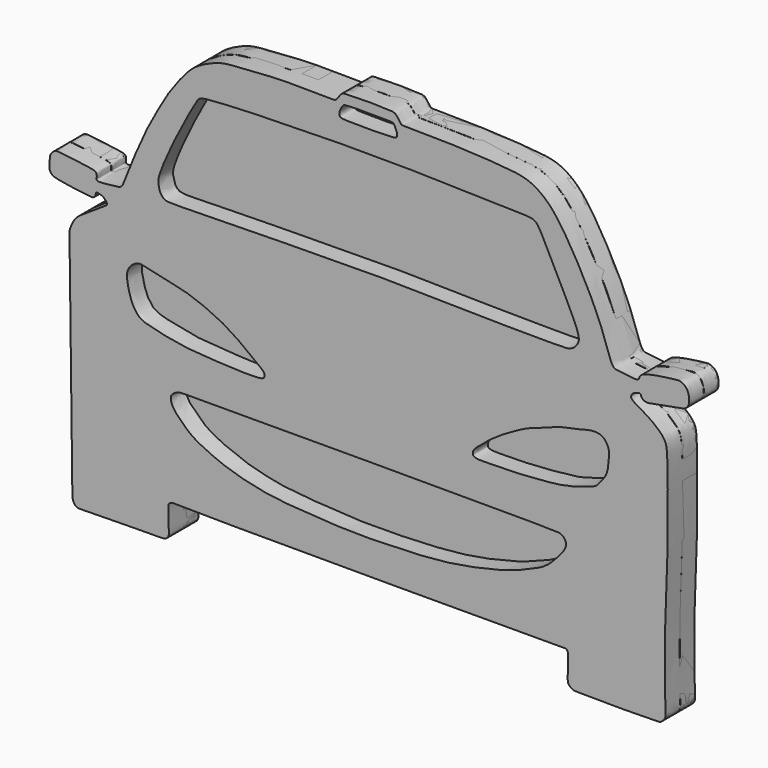
from build123d import *

# Parameters (mm, degrees)
F1_DEPTH = 10
F3_DEPTH = 5


# Not quite as in the source:
# - the dataset's text gives a spline's control points without its knots; the knots are read off the source's solid


with BuildPart() as f1:
    # F0 (on Front) → F1 (new body)
    with BuildSketch(Plane.XZ):
        with BuildLine():
            add(Edge.make_bspline(
                [(-21.2726220489, 56.9635778666), (-18.9281210434, 56.9386434726), (-13.6200187911, 56.9350553762), (-12.4767039382, 56.8796603206), (-11.0844689446, 59.0635225696), (-10.0407495433, 59.5178063954), (2.4345859918, 59.518579453), (3.2763047499, 59.1466182179), (3.9763116908, 58.8890525048), (5.0929181479, 56.9335783544), (5.904101681, 56.724426004), (15.4186256689, 56.7606694424), (22.415242163, 56.5636878104), (29.6627233817, 56.1516039707), (36.4134224992, 55.6653181625), (40.7970991211, 54.6157339048), (45.7371435577, 51.1119020349), (50.2355062798, 44.586092306), (55.3245831337, 35.7107979243), (59.9788649432, 25.7843744812), (62.2274911548, 17.8785094194), (63.6873972743, 17.2156075688), (66.8512747735, 16.9837572481), (69.6520031247, 16.5690870165), (69.8806873946, 17.6725077821), (70.4097864802, 18.6062553039), (74.7105095588, 19.635285385), (79.2407912013, 20.1558018394), (81.1270530867, 20.4040771455), (82.9879359908, 19.1249872852), (83.5930078541, 16.4735751448), (82.9736764331, 13.9928114241), (79.4258491754, 13.6783873856), (73.7801155733, 12.3750310277), (71.463650212, 12.0317762657), (70.2694302292, 12.9854799945), (70.3246556827, 14.0053639175), (68.0167941293, 13.3915679245), (67.2779003031, 11.8146832667), (69.6477321499, 10.3935148412), (73.5277584139, 8.2297653036), (76.3688101278, 5.512225397), (77.553760652, 3.3461910931), (77.5530453586, -6.9270704509), (77.6729301989, -20.5721617917), (76.8765812567, -35.8181398753), (76.7627137917, -48.5519759849), (76.7695297304, -57.1100262171), (77.1198420733, -60.9187955099), (76.7184740375, -61.9661008778), (75.7188165531, -62.9575649684), (74.57226928, -63.2191940943), (52.313578017, -63.2602932478), (51.7170076075, -62.9598727868), (50.8037103143, -62.3515989217), (50.4461995219, -61.6734356735), (50.3566400858, -60.312061393), (50.496949856, -55.8709343448), (50.5163145323, -54.6497774244), (50.2924540607, -53.7307567814), (48.869529547, -53.7163267319), (48.4763551332, -53.8276018998), (-54.7929577116, -54.0161919263), (-56.6230034085, -53.5809102698), (-57.8696673343, -53.9463225485), (-57.9690717545, -54.8661327531), (-57.9613761424, -55.8743450215), (-57.78340253, -61.3734469783), (-57.906912999, -61.8656330337), (-58.3760760652, -62.8292128086), (-59.8541306513, -63.0064316834), (-61.119934638, -62.9784770213), (-81.3057995002, -63.1510879072), (-81.9270637775, -63.3194642105), (-83.0199574255, -63.1533789577), (-83.5677741934, -62.4923589555), (-84.0399677683, -61.4612616226), (-84.1109783652, -59.7084531519), (-84.0532967239, -54.3188819205), (-84.2059386301, -39.499846326), (-84.5404697297, -24.4846736289), (-84.6842054736, -4.2904268447), (-84.9727713877, 1.6036548675), (-84.6122092098, 3.1704690828), (-83.4970696269, 5.5484038074), (-81.9083921978, 6.9864352173), (-78.9297296369, 8.7724944135), (-76.6131468274, 10.515826782), (-74.6581214491, 11.5553240796), (-74.6426954546, 12.1225788132), (-75.0666632198, 12.9146555158), (-76.0348664394, 13.591346412), (-77.0102810448, 13.8064368612), (-77.5889687922, 13.8905870458), (-77.7555570585, 13.1194908993), (-77.8783275013, 12.5728149948), (-78.6488107317, 12.2151925415), (-79.8144730652, 12.3421801098), (-87.754645938, 13.3273577072), (-89.7442692365, 14.0688538765), (-90.3708386486, 15.3126490716), (-90.2186233578, 16.685187407), (-90.2011514391, 18.346575344), (-89.7260237086, 19.3326468169), (-88.6939660926, 20.2602979581), (-87.0893708951, 20.1537941529), (-84.2859429545, 19.7755893206), (-80.7326560197, 19.3338400413), (-78.0451968926, 18.9618621225), (-77.4081568708, 18.4038525579), (-77.3850675835, 17.3042629393), (-77.6174256376, 16.6571560893), (-76.0385293662, 16.5012085027), (-73.6413404779, 16.9400882023), (-70.68829264, 16.9931303492), (-70.0675967459, 18.6874870731), (-68.5910153059, 22.5032449084), (-64.2564188952, 32.8703041995), (-60.8249096081, 38.9385754701), (-57.8737837643, 44.1866083784), (-54.2854935401, 48.980022304), (-51.057079458, 52.4849366267), (-47.5395759836, 54.3378193748), (-43.7334971009, 55.8696843536), (-39.8300474742, 56.2378976637), (-32.3869709385, 56.8090194268), (-25.0928653652, 57.0502633666), (-22.9556034711, 56.9814768232), (-21.2726220489, 56.9635778666)],
                knots=[0, 0, 0, 0, 0.012004279, 0.0166060931, 0.0229256448, 0.0281319073, 0.0432673507, 0.0475023634, 0.0509727754, 0.0572163817, 0.0610794225, 0.0740101169, 0.0861690954, 0.0977510892, 0.1089672006, 0.1180487717, 0.1284009233, 0.1405580043, 0.1544730395, 0.1693317649, 0.1811779425, 0.1860858482, 0.1939223982, 0.2008529986, 0.2047123352, 0.2088215587, 0.2178047105, 0.2273021586, 0.2330687556, 0.2391473012, 0.2462002175, 0.2524569245, 0.2602934775, 0.2709255551, 0.2774471417, 0.2823111627, 0.2858315267, 0.2918561735, 0.2968070097, 0.3033862826, 0.3128308377, 0.3212326352, 0.3276933936, 0.3410856773, 0.3575651839, 0.3745816846, 0.3901986349, 0.4028768542, 0.4109320455, 0.4153236614, 0.4199204056, 0.4252759381, 0.4455314568, 0.4496448447, 0.4537977426, 0.4574222191, 0.4625115378, 0.4716783043, 0.4766263187, 0.4803465727, 0.4847295197, 0.4896306962, 0.533369126, 0.5407513134, 0.5447167402, 0.5484229444, 0.5531979597, 0.5632282462, 0.5665861336, 0.5706917749, 0.5754184792, 0.5812469368, 0.6004920236, 0.6046145035, 0.6087124203, 0.6126751413, 0.6171358015, 0.6225679613, 0.63233332, 0.648837342, 0.6664896516, 0.6859542941, 0.6959514414, 0.7011876078, 0.7079812388, 0.7143927888, 0.722400922, 0.7300977008, 0.7361918541, 0.7390107332, 0.7429853976, 0.7477261765, 0.7520874229, 0.7550056805, 0.7585574057, 0.7618058195, 0.7653503812, 0.7701326602, 0.7823994269, 0.7887832793, 0.7934012506, 0.7985126711, 0.8040633285, 0.8085537263, 0.8133764402, 0.8186789388, 0.825980184, 0.8344524837, 0.8414202702, 0.845081123, 0.8495126559, 0.8525366189, 0.8572853902, 0.8644418039, 0.8715383863, 0.8766814644, 0.8853463362, 0.8999599019, 0.9116536105, 0.9221471426, 0.9327623493, 0.9421527591, 0.9507359878, 0.9593353611, 0.9678654751, 0.9798461294, 0.9913828237, 1, 1, 1, 1], degree=3))
        make_face()
        with BuildLine():
            add(Edge.make_bspline(
                [(-53.1355589628, -26.5916269273), (-53.6976261616, -26.5964024078), (-54.7832478549, -26.5807781137), (-56.0233124859, -26.9576088353), (-57.4068308066, -28.0020644289), (-57.3223140239, -29.6697594393), (-56.2385573069, -31.6264394585), (-54.574722627, -33.1702280567), (-51.9418061953, -36.0076064052), (-46.3671903717, -38.7239087732), (-40.4685519219, -41.1333015304), (-30.5424899792, -43.4525625201), (-22.3232735976, -43.9772319436), (-9.2867544557, -44.9236923228), (1.1993285628, -44.6889216672), (10.8839715562, -44.3309053124), (18.6551069165, -43.6032529515), (25.152762993, -42.4398108365), (33.9704603673, -40.491225791), (41.4046227696, -37.4482689073), (45.1840875394, -35.5126166261), (48.7429680129, -31.4913886381), (50.0565149772, -29.5272469574), (49.9175813156, -27.8968660654), (48.7318024113, -26.7300201474), (46.5449775529, -26.4557090204), (23.193318347, -26.5842552421), (9.0526969316, -26.3970421968), (-18.087431957, -26.564441631), (-43.2680076928, -26.5233169993), (-50.7705705235, -26.5249350214), (-52.5033477422, -26.5862554834), (-53.1355589628, -26.5916269273)],
                knots=[0, 0, 0, 0, 0.0171126114, 0.0323888607, 0.0490571733, 0.0654263189, 0.0851073726, 0.1051342912, 0.1311088377, 0.1640384324, 0.1984074172, 0.2404194754, 0.2795803906, 0.327564471, 0.3715811823, 0.4130663176, 0.4500873651, 0.4843764852, 0.5249027849, 0.5626102853, 0.5904227705, 0.6209881894, 0.6412442562, 0.6572639193, 0.6729750723, 0.6916365136, 0.754333791, 0.8082138255, 0.8780108631, 0.9459992677, 0.9807517945, 1, 1, 1, 1], degree=3))
        make_face(mode=Mode.SUBTRACT)
        with BuildLine():
            add(Edge.make_bspline(
                [(-69.1952109337, -3.0402038246), (-69.1424189669, -2.4984055481), (-68.8148194617, -1.2736033989), (-67.3949290593, 0.0820577786), (-65.9181183156, 0.7428462405), (-64.1545786431, 0.3387350994), (-62.9742030562, -0.033511915), (-60.7451687242, -0.4389260423), (-57.8760916225, -1.1231888825), (-52.7883947077, -2.0536024885), (-46.104853418, -4.7271514053), (-41.0694692542, -7.3915702461), (-35.8487768109, -11.2367185072), (-33.1296719116, -13.4064907124), (-31.8055118753, -14.4905497602), (-31.8378797306, -15.6377541782), (-33.1632163341, -16.508413198), (-43.5009558887, -15.9749025925), (-53.3210116898, -15.5878530618), (-62.1417127348, -13.6788598688), (-66.4403055716, -12.4826132699), (-68.5090453278, -8.0609543999), (-69.1293631943, -4.7019781284), (-69.2454605096, -3.5559098175), (-69.1952109337, -3.0402038246)],
                knots=[0, 0, 0, 0, 0.0320196923, 0.065499859, 0.0958165204, 0.1273607104, 0.1545542305, 0.1900549915, 0.2315564976, 0.2866521737, 0.3516113788, 0.4105079055, 0.4720579233, 0.5173564411, 0.5473202344, 0.5700042289, 0.5960155031, 0.6718077521, 0.7521620586, 0.8237759166, 0.8730492088, 0.9247389547, 0.9695223335, 1, 1, 1, 1], degree=3))
        make_face(mode=Mode.SUBTRACT)
        with BuildLine():
            add(Edge.make_bspline(
                [(25.1084696501, -14.1660654917), (25.6540619714, -13.4663718217), (28.3062823201, -11.2834146748), (31.3859609659, -8.9219493596), (35.3388643066, -6.6977252539), (39.2542756594, -4.4164967342), (43.1290163399, -3.3095281506), (48.4797774939, -1.0608922569), (52.4127941876, -0.5765318964), (56.2564842473, 0.6546022799), (58.4231026966, 0.6713662683), (59.8728002993, 0.29472284), (60.8040810028, -0.7587122488), (61.5376427074, -1.9171484482), (61.6715250629, -3.6553191141), (61.4218124054, -6.9657615397), (60.7891094279, -9.0375031972), (59.4457459168, -10.6461906832), (58.1530864339, -12.4844272336), (54.8304034955, -13.4251367256), (49.5935068191, -15.1942662854), (42.1931968703, -15.7011666479), (35.5458249636, -16.2798963427), (28.2040253207, -16.2662368017), (26.0113076396, -16.359483591), (24.6366653823, -15.9146003071), (24.6885594166, -14.972701183), (24.8435275541, -14.5058398989), (25.1084696501, -14.1660654917)],
                knots=[0, 0, 0, 0, 0.0440680216, 0.0886155606, 0.1349438291, 0.1810566843, 0.2253393957, 0.2774722033, 0.3218816033, 0.3652691177, 0.3971182977, 0.4229159769, 0.4482939477, 0.4732133666, 0.5018868598, 0.5417532018, 0.5740494224, 0.6050621963, 0.6368234352, 0.6761853188, 0.727842775, 0.787136851, 0.8454760723, 0.9039954673, 0.9363768685, 0.9598413388, 0.9786003696, 1, 1, 1, 1], degree=3))
        make_face(mode=Mode.SUBTRACT)
        with BuildLine():
            add(Edge.make_bspline(
                [(-60.449089855, 23.4657637775), (-59.7268025829, 25.9499990787), (-55.0486740257, 36.2434537738), (-50.5332078122, 44.0234861939), (-49.6507117627, 45.4153832966), (-46.8182608482, 46.101614448), (-27.1444997198, 46.8410624017), (-6.2434253638, 47.1236015085), (10.4093497943, 47.0115942379), (24.7820490758, 46.4248668332), (37.2365310555, 46.3920094353), (41.3157920888, 46.1061273348), (42.5430313027, 44.7082181192), (44.4128868997, 41.0993496919), (51.7262229522, 26.6293422844), (53.4288483565, 22.3410559411), (53.4876735773, 20.6668200126), (52.6559620042, 19.2659246588), (51.0466721601, 18.1077877285), (47.1693282378, 17.9605728629), (20.0961842353, 18.1762825131), (1.4343835567, 18.7276400432), (-16.161689366, 18.42452892), (-33.2311431388, 18.2960955003), (-50.942296833, 17.9245371375), (-57.2257493926, 17.7592393643), (-58.9496006688, 17.9445631908), (-60.3064745533, 19.2022800159), (-60.7305795333, 21.5274846067), (-60.7294395974, 22.5015286955), (-60.449089855, 23.4657637775)],
                knots=[0, 0, 0, 0, 0.0485545096, 0.0880602762, 0.1025427788, 0.1219632464, 0.178705447, 0.2405848743, 0.2932012218, 0.3433031999, 0.3890983759, 0.4137241752, 0.4292712749, 0.4554512066, 0.5084918276, 0.5364774142, 0.5518269012, 0.5679089262, 0.5848675339, 0.6089555856, 0.6757754093, 0.7348302827, 0.7881140486, 0.8430319301, 0.8980602928, 0.9293307078, 0.9452000073, 0.962029116, 0.9811539746, 1, 1, 1, 1], degree=3))
        make_face(mode=Mode.SUBTRACT)
        with BuildLine():
            add(Edge.make_bspline(
                [(-11.2904524431, 55.1297776401), (-11.1115287097, 55.519461541), (-10.5980162373, 56.4650279611), (-9.6120436313, 56.8741720608), (1.7409666504, 56.727890187), (3.0280762308, 56.7364002279), (3.5493267653, 55.9093014316), (4.3759679528, 54.0300009265), (3.740707024, 53.2219744216), (2.3311488499, 53.0245501687), (-10.0860616691, 52.8912859084), (-11.4776807276, 53.2978044687), (-11.6054331302, 54.3278758953), (-11.4361285139, 54.8125049202), (-11.2904524431, 55.1297776401)],
                knots=[0, 0, 0, 0, 0.0658482757, 0.1265141893, 0.3172156325, 0.381186547, 0.4333981353, 0.5132132762, 0.5618033335, 0.6303139517, 0.8310266809, 0.8958004356, 0.9463876709, 1, 1, 1, 1], degree=3))
        make_face(mode=Mode.SUBTRACT)
    extrude(amount=F1_DEPTH)


with BuildPart() as f3:
    # F2 (on Front) → F3 (new body)
    with BuildSketch(Plane.XZ):
        with BuildLine():
            add(Edge.make_bspline(
                [(-21.2726220489, 56.9635778666), (-18.9281210434, 56.9386434726), (-13.6200187911, 56.9350553762), (-12.4767039382, 56.8796603206), (-11.0844689446, 59.0635225696), (-10.0407495433, 59.5178063954), (2.4345859918, 59.518579453), (3.2763047499, 59.1466182179), (3.9763116908, 58.8890525048), (5.0929181479, 56.9335783544), (5.904101681, 56.724426004), (15.4186256689, 56.7606694424), (22.415242163, 56.5636878104), (29.6627233817, 56.1516039707), (36.4134224992, 55.6653181625), (40.7970991211, 54.6157339048), (45.7371435577, 51.1119020349), (50.2355062798, 44.586092306), (55.3245831337, 35.7107979243), (59.9788649432, 25.7843744812), (62.2274911548, 17.8785094194), (63.6873972743, 17.2156075688), (66.8512747735, 16.9837572481), (69.6520031247, 16.5690870165), (69.8806873946, 17.6725077821), (70.4097864802, 18.6062553039), (74.7105095588, 19.635285385), (79.2407912013, 20.1558018394), (81.1270530867, 20.4040771455), (82.9879359908, 19.1249872852), (83.5930078541, 16.4735751448), (82.9736764331, 13.9928114241), (79.4258491754, 13.6783873856), (73.7801155733, 12.3750310277), (71.463650212, 12.0317762657), (70.2694302292, 12.9854799945), (70.3246556827, 14.0053639175), (68.0167941293, 13.3915679245), (67.2779003031, 11.8146832667), (69.6477321499, 10.3935148412), (73.5277584139, 8.2297653036), (76.3688101278, 5.512225397), (77.553760652, 3.3461910931), (77.5530453586, -6.9270704509), (77.6729301989, -20.5721617917), (76.8765812567, -35.8181398753), (76.7627137917, -48.5519759849), (76.7695297304, -57.1100262171), (77.1198420733, -60.9187955099), (76.7184740375, -61.9661008778), (75.7188165531, -62.9575649684), (74.57226928, -63.2191940943), (52.313578017, -63.2602932478), (51.7170076075, -62.9598727868), (50.8037103143, -62.3515989217), (50.4461995219, -61.6734356735), (50.3566400858, -60.312061393), (50.496949856, -55.8709343448), (50.5163145323, -54.6497774244), (50.2924540607, -53.7307567814), (48.869529547, -53.7163267319), (48.4763551332, -53.8276018998), (-54.7929577116, -54.0161919263), (-56.6230034085, -53.5809102698), (-57.8696673343, -53.9463225485), (-57.9690717545, -54.8661327531), (-57.9613761424, -55.8743450215), (-57.78340253, -61.3734469783), (-57.906912999, -61.8656330337), (-58.3760760652, -62.8292128086), (-59.8541306513, -63.0064316834), (-61.119934638, -62.9784770213), (-81.3057995002, -63.1510879072), (-81.9270637775, -63.3194642105), (-83.0199574255, -63.1533789577), (-83.5677741934, -62.4923589555), (-84.0399677683, -61.4612616226), (-84.1109783652, -59.7084531519), (-84.0532967239, -54.3188819205), (-84.2059386301, -39.499846326), (-84.5404697297, -24.4846736289), (-84.6842054736, -4.2904268447), (-84.9727713877, 1.6036548675), (-84.6122092098, 3.1704690828), (-83.4970696269, 5.5484038074), (-81.9083921978, 6.9864352173), (-78.9297296369, 8.7724944135), (-76.6131468274, 10.515826782), (-74.6581214491, 11.5553240796), (-74.6426954546, 12.1225788132), (-75.0666632198, 12.9146555158), (-76.0348664394, 13.591346412), (-77.0102810448, 13.8064368612), (-77.5889687922, 13.8905870458), (-77.7555570585, 13.1194908993), (-77.8783275013, 12.5728149948), (-78.6488107317, 12.2151925415), (-79.8144730652, 12.3421801098), (-87.754645938, 13.3273577072), (-89.7442692365, 14.0688538765), (-90.3708386486, 15.3126490716), (-90.2186233578, 16.685187407), (-90.2011514391, 18.346575344), (-89.7260237086, 19.3326468169), (-88.6939660926, 20.2602979581), (-87.0893708951, 20.1537941529), (-84.2859429545, 19.7755893206), (-80.7326560197, 19.3338400413), (-78.0451968926, 18.9618621225), (-77.4081568708, 18.4038525579), (-77.3850675835, 17.3042629393), (-77.6174256376, 16.6571560893), (-76.0385293662, 16.5012085027), (-73.6413404779, 16.9400882023), (-70.68829264, 16.9931303492), (-70.0675967459, 18.6874870731), (-68.5910153059, 22.5032449084), (-64.2564188952, 32.8703041995), (-60.8249096081, 38.9385754701), (-57.8737837643, 44.1866083784), (-54.2854935401, 48.980022304), (-51.057079458, 52.4849366267), (-47.5395759836, 54.3378193748), (-43.7334971009, 55.8696843536), (-39.8300474742, 56.2378976637), (-32.3869709385, 56.8090194268), (-25.0928653652, 57.0502633666), (-22.9556034711, 56.9814768232), (-21.2726220489, 56.9635778666)],
                knots=[0, 0, 0, 0, 0.012004279, 0.0166060931, 0.0229256448, 0.0281319073, 0.0432673507, 0.0475023634, 0.0509727754, 0.0572163817, 0.0610794225, 0.0740101169, 0.0861690954, 0.0977510892, 0.1089672006, 0.1180487717, 0.1284009233, 0.1405580043, 0.1544730395, 0.1693317649, 0.1811779425, 0.1860858482, 0.1939223982, 0.2008529986, 0.2047123352, 0.2088215587, 0.2178047105, 0.2273021586, 0.2330687556, 0.2391473012, 0.2462002175, 0.2524569245, 0.2602934775, 0.2709255551, 0.2774471417, 0.2823111627, 0.2858315267, 0.2918561735, 0.2968070097, 0.3033862826, 0.3128308377, 0.3212326352, 0.3276933936, 0.3410856773, 0.3575651839, 0.3745816846, 0.3901986349, 0.4028768542, 0.4109320455, 0.4153236614, 0.4199204056, 0.4252759381, 0.4455314568, 0.4496448447, 0.4537977426, 0.4574222191, 0.4625115378, 0.4716783043, 0.4766263187, 0.4803465727, 0.4847295197, 0.4896306962, 0.533369126, 0.5407513134, 0.5447167402, 0.5484229444, 0.5531979597, 0.5632282462, 0.5665861336, 0.5706917749, 0.5754184792, 0.5812469368, 0.6004920236, 0.6046145035, 0.6087124203, 0.6126751413, 0.6171358015, 0.6225679613, 0.63233332, 0.648837342, 0.6664896516, 0.6859542941, 0.6959514414, 0.7011876078, 0.7079812388, 0.7143927888, 0.722400922, 0.7300977008, 0.7361918541, 0.7390107332, 0.7429853976, 0.7477261765, 0.7520874229, 0.7550056805, 0.7585574057, 0.7618058195, 0.7653503812, 0.7701326602, 0.7823994269, 0.7887832793, 0.7934012506, 0.7985126711, 0.8040633285, 0.8085537263, 0.8133764402, 0.8186789388, 0.825980184, 0.8344524837, 0.8414202702, 0.845081123, 0.8495126559, 0.8525366189, 0.8572853902, 0.8644418039, 0.8715383863, 0.8766814644, 0.8853463362, 0.8999599019, 0.9116536105, 0.9221471426, 0.9327623493, 0.9421527591, 0.9507359878, 0.9593353611, 0.9678654751, 0.9798461294, 0.9913828237, 1, 1, 1, 1], degree=3))
        make_face()
    extrude(amount=F3_DEPTH)


solid = Compound([f1.part, f3.part])
